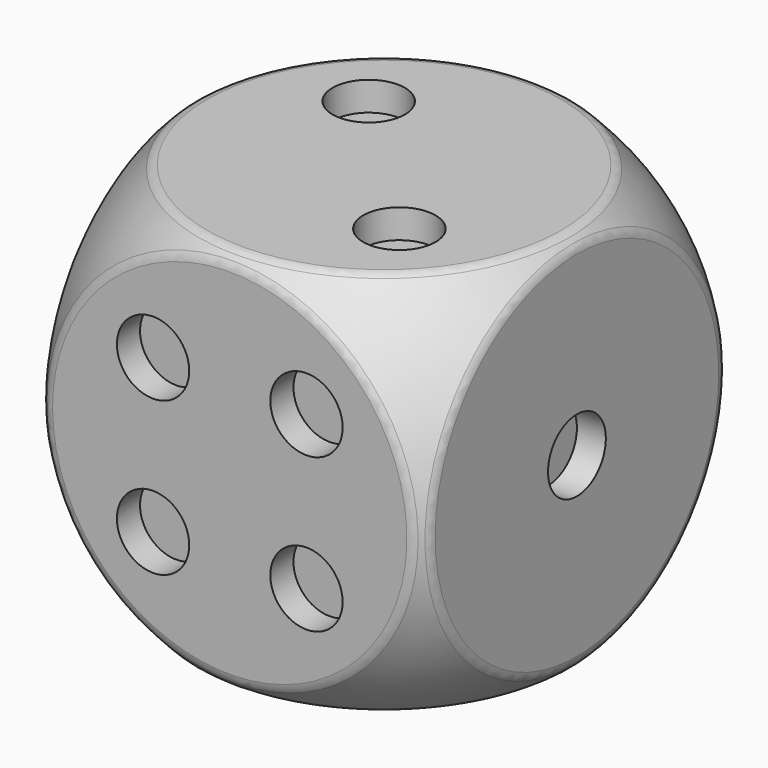
from build123d import *

# Parameters (mm, degrees)
F0_W          = 16
F0_H          = 16
F1_DEPTH      = 8
F4_R          = 0.5
F5_R          = 1.5
F6_DEPTH      = 1.2
F7_R          = 1.5
F8_DEPTH      = 1.2
F9_R          = 1.5
F10_DEPTH     = 1.2
F11_R         = 1.5
F12_DEPTH     = 1.2
F13_R         = 1.5
F14_DEPTH     = 1.2
F15_TEXT_SIZE = 5.5555555556
F16_DEPTH     = 3.4


# Not quite as in the source:
# - Text() gives the source's letters only with a copy of the font that has no kerning and outlines rounded to 1/6400 em; it was checked with that copy


with BuildPart() as f1:
    # F0 (on Top) → F1 (new body, symmetric)
    with BuildSketch(Plane.XY):
        Rectangle(F0_W, F0_H)
    extrude(amount=F1_DEPTH, both=True)

    # F2 (on Top) → F3 (revolve, cut)
    with BuildSketch(Plane.XY):
        with BuildLine():
            ThreePointArc((0, -11), (-11, 0), (0, 11))
            Line((0, 11), (0, 18.8876076052))
            ThreePointArc((0, 18.8876076052), (-18.8876076052, 0), (0, -18.8876076052))
            Line((0, -18.8876076052), (0, -11))
        make_face()
    revolve(axis=Axis((0, -2.4417540575, 0), (0, -1, 0)), mode=Mode.SUBTRACT)

    # F4
    f4_edges = [f1.edges().sort_by_distance(p)[0] for p in [
        (0, 7.549834, 8),
        (7.549834, -8, 0),
        (-8, 0, -7.549834),
        (-8, 0, 7.549834),
        (8, 0, -7.549834),
        (7.549834, 8, 0),
        (0, 7.549834, -8),
    ]]
    fillet(f4_edges, radius=F4_R)

    # F5 (on face) → F6 (cut)
    with BuildSketch(Plane.XY.offset(8)):
        with Locations((-3.1819805153, 3.1819805153)):
            Circle(F5_R)
        with Locations((3.1819805153, -3.1819805153)):
            Circle(F5_R)
    extrude(amount=-F6_DEPTH, mode=Mode.SUBTRACT)

    # F7 (on face) → F8 (cut)
    with BuildSketch(Plane.YZ.offset(8)):
        Circle(F7_R)
    extrude(amount=-F8_DEPTH, mode=Mode.SUBTRACT)

    # F9 (on face) → F10 (cut)
    with BuildSketch(Plane(origin=(0, 0, -8), x_dir=(1, 0, 0), z_dir=(0, 0, -1))):
        with Locations((-3.1819805153, 3.1819805153)):
            Circle(F9_R)
        Circle(F9_R)
        with Locations((3.1819805153, 3.1819805153)):
            Circle(F9_R)
        with Locations((3.1819805153, -3.1819805153)):
            Circle(F9_R)
        with Locations((-3.1819805153, -3.1819805153)):
            Circle(F9_R)
    extrude(amount=-F10_DEPTH, mode=Mode.SUBTRACT)

    # F11 (on face) → F12 (cut)
    with BuildSketch(Plane.XZ.offset(8)):
        with Locations((-3.1819805153, 3.1819805153)):
            Circle(F11_R)
        with Locations((3.1819805153, 3.1819805153)):
            Circle(F11_R)
        with Locations((3.1819805153, -3.1819805153)):
            Circle(F11_R)
        with Locations((-3.1819805153, -3.1819805153)):
            Circle(F11_R)
    extrude(amount=-F12_DEPTH, mode=Mode.SUBTRACT)

    # F13 (on face) → F14 (cut)
    with BuildSketch(Plane(origin=(0, 8, 0), x_dir=(-1, 0, 0), z_dir=(0, 1, 0))):
        with Locations((-3.1660905034, 3.1660905034)):
            Circle(F13_R)
        Circle(F13_R)
        with Locations((3.1978705273, -3.1978705273)):
            Circle(F13_R)
    extrude(amount=-F14_DEPTH, mode=Mode.SUBTRACT)

    # F15 (on face) → F16 (cut)
    with BuildSketch(Plane(origin=(-8, 0, 0), x_dir=(0, -1, 0), z_dir=(-1, 0, 0))):
        with Locations((-6.5655284949, -2)):
            Text('APES', F15_TEXT_SIZE, font='Open Sans', text_align=(TextAlign.LEFT, TextAlign.BOTTOM))
    extrude(amount=-F16_DEPTH, mode=Mode.SUBTRACT)


solid = f1.part
